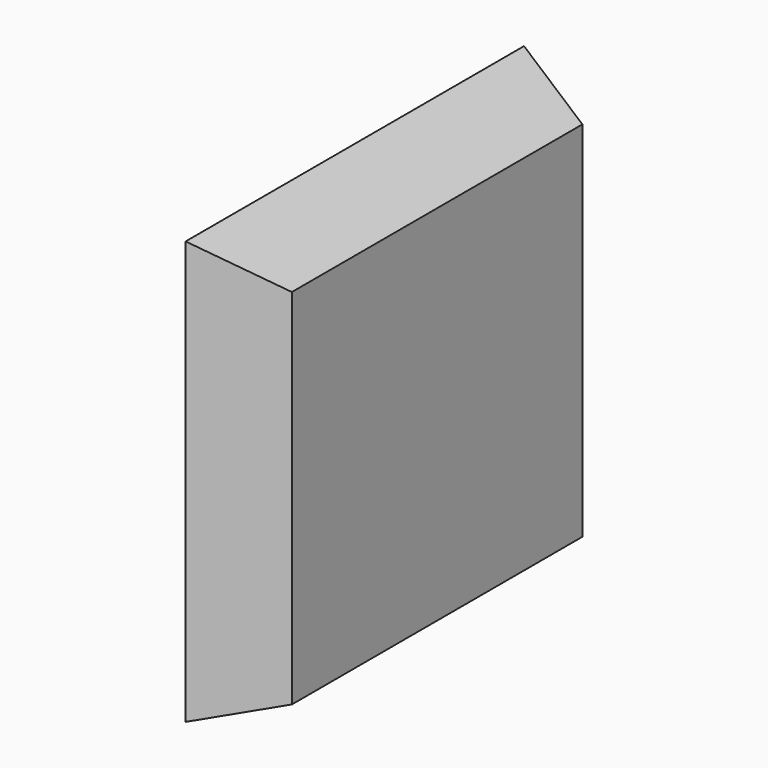
from build123d import *

# Parameters (mm, degrees)
F0_W        = 130.2845291793
F0_H        = 130.2845217288
F1_DEPTH    = 25
F2_T1_DEPTH = 272.8343581663
F2_T3_DEPTH = 272.8343507158


# Not quite as in the source:
# - a fillet or chamfer that OpenCascade refuses, or shapes differently, is made with other operations: its cross-section is extruded or revolved along the edge and cut away or added


with BuildPart() as f1:
    # F0 (on Right) → F1 (new body)
    with BuildSketch(Plane.YZ):
        with Locations((-37.4803263694, 21.2906058878)):
            Rectangle(F0_W, F0_H)
    extrude(amount=F1_DEPTH)

    # F2: chamfer of 10 x 27.4747741945 on 4 edges, made by hand

    # F2_s2 → F2_t1 (cut)
    with BuildSketch(Plane.XZ.offset(-98.9368527138)):
        Polygon((-2.4747741945, -43.8516549766), (25, -33.8516549766), (25, -43.8516549766), align=None)
        Polygon((-2.4747741945, 86.4328667521), (25, 76.4328667521), (25, 86.4328667521), align=None)
    extrude(amount=F2_T1_DEPTH, mode=Mode.SUBTRACT)

    # F2_s4 → F2_t3 (cut)
    with BuildSketch(Plane.XY.offset(-115.1265694701)):
        Polygon((-2.4747741945, -102.6225909591), (25, -92.6225909591), (25, -102.6225909591), align=None)
        Polygon((-2.4747741945, 27.6619382203), (25, 17.6619382203), (25, 27.6619382203), align=None)
    extrude(amount=F2_T3_DEPTH, mode=Mode.SUBTRACT)


solid = f1.part
